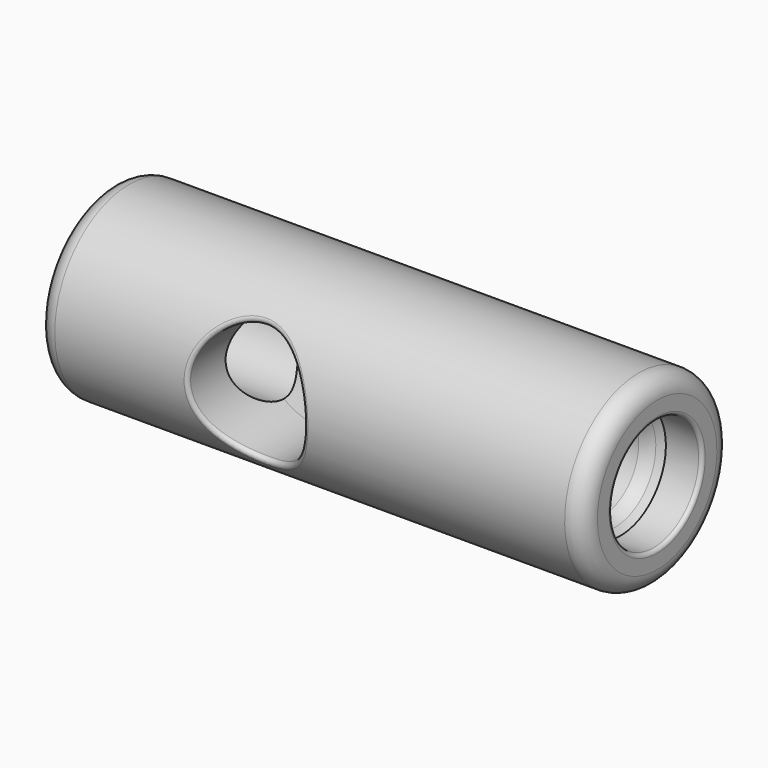
from build123d import *

# Parameters (mm, degrees)
F2_R          = 1
F3_R          = 3.2
F4_DEPTH      = 25.4
F4_DEPTH_BACK = 25.4
F5_R          = 0.2


with BuildPart() as f1:
    # F0 (on Front) → F1 (revolve)
    with BuildSketch(Plane.XZ):
        Polygon((-15, 5.1), (-15, 3.1), (-13, 3.1), (-12.4, 2.5), (12.4, 2.5), (13, 3.1), (15, 3.1), (15, 5.1), align=None)
    revolve(axis=Axis((0, 0, 0), (1, 0, 0)))

    # F2
    f2_edges = [f1.edges().sort_by_distance(p)[0] for p in [
        (15, 0, -5.1),
        (-15, 0, -5.1),
        (0, 0, 5.1),
        (-12.4, 0, -2.5),
        (12.4, 0, -2.5),
        (0, 0, 2.5),
    ]]
    fillet(f2_edges, radius=F2_R)

    # F3 (on Front) → F4 (cut, two sides)
    with BuildSketch(Plane.XZ) as f4_sk:
        with Locations((-3.5, 0)):
            Circle(F3_R)
    extrude(amount=-F4_DEPTH, mode=Mode.SUBTRACT)
    extrude(f4_sk.sketch, amount=F4_DEPTH_BACK, mode=Mode.SUBTRACT)

    # F5
    f5_edges = [f1.edges().sort_by_distance(p)[0] for p in [
        (-6.7, -5.1, 0),
        (-6.7, 5.1, 0),
        (15, 0, -3.1),
        (-15, 0, -3.1),
    ]]
    fillet(f5_edges, radius=F5_R)


solid = f1.part
